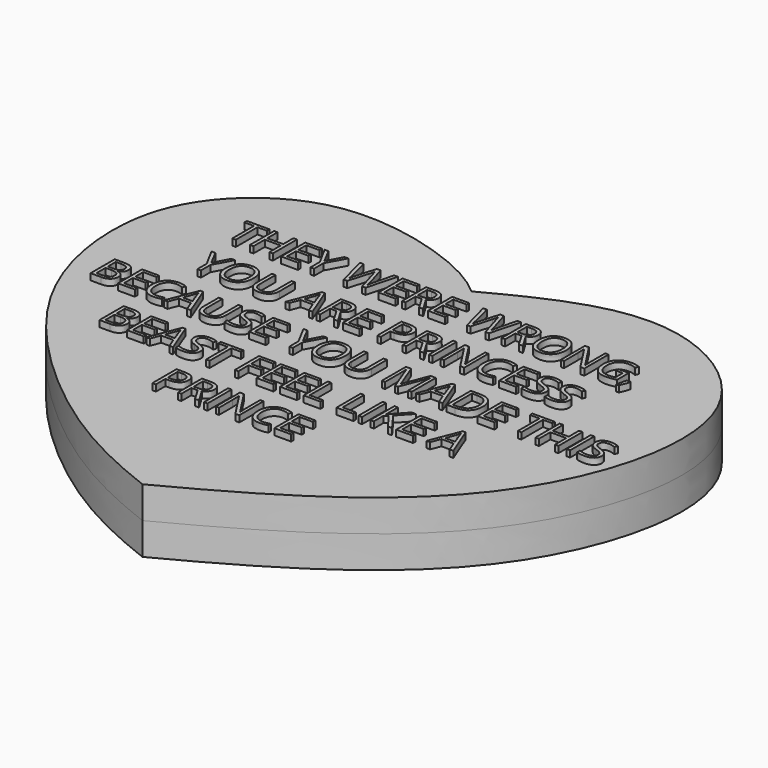
from build123d import *

# Parameters (mm, degrees)
F2_DEPTH     = 5
F1_TEXT_SIZE = 6.6096924944
F3_DEPTH     = 6


# Not quite as in the source:
# - Text() gives the source's letters only with a copy of the font that has no kerning and outlines rounded to 1/6400 em; it was checked with that copy


with BuildPart() as f2:
    # F0 (on Top) → F2 (new body, symmetric)
    with BuildSketch(Plane.XY):
        with BuildLine():
            add(Edge.make_bspline(
                [(49.6034175158, 70.3383758664), (57.4255755938, 74.4701894092), (72.777071302, 82.1686280864), (98.5809075936, 66.4625184016), (89.6533310415, 28.6744955736), (66.9245487128, 14.178657317), (50.0742010772, 5.4191295058)],
                knots=[0, 0, 0, 0, 0.2245214689, 0.4410611027, 0.6922062561, 1, 1, 1, 1], degree=3))
            add(Edge.make_bspline(
                [(49.6034175158, 70.3383758664), (47.4339338141, 72.2192165566), (41.0433747036, 76.0012562734), (22.277013048, 80.0594704424), (7.7702176976, 69.6318815381), (3.9007087353, 55.4213262189), (8.818104806, 34.6134665552), (31.3463892668, 13.6516026811), (43.7721535607, 7.8800658319), (50.0742010772, 5.4191295058)],
                knots=[0, 0, 0, 0, 0.106242303, 0.2507252939, 0.3862136345, 0.5102499506, 0.6625335349, 0.8471651701, 1, 1, 1, 1], degree=3))
        make_face()
    extrude(amount=F2_DEPTH, both=True)

    # F1 (on Top) → F3 (join)
    with BuildSketch(Plane.XY):
        with Locations((17.7022512533, 61.5221194269)):
            Text('THEY WERE WRONG,', F1_TEXT_SIZE, font='Open Sans', text_align=(TextAlign.LEFT, TextAlign.BOTTOM))
        with Locations((19.4197385374, 52.5329376346)):
            Text('YOU ARE PRINCESS', F1_TEXT_SIZE, font='Open Sans', text_align=(TextAlign.LEFT, TextAlign.BOTTOM))
        with Locations((10.832302117, 43.5437558422)):
            Text('BECAUSE YOU MADE THIS', F1_TEXT_SIZE, font='Open Sans', text_align=(TextAlign.LEFT, TextAlign.BOTTOM))
        with Locations((19.4197385374, 34.5545740498)):
            Text('BEAST FEEL LIKE A', F1_TEXT_SIZE, font='Open Sans', text_align=(TextAlign.LEFT, TextAlign.BOTTOM))
        with Locations((34.8771240942, 25.5653922575)):
            Text('PRINCE', F1_TEXT_SIZE, font='Open Sans', text_align=(TextAlign.LEFT, TextAlign.BOTTOM))
    extrude(amount=F3_DEPTH)


solid = f2.part
